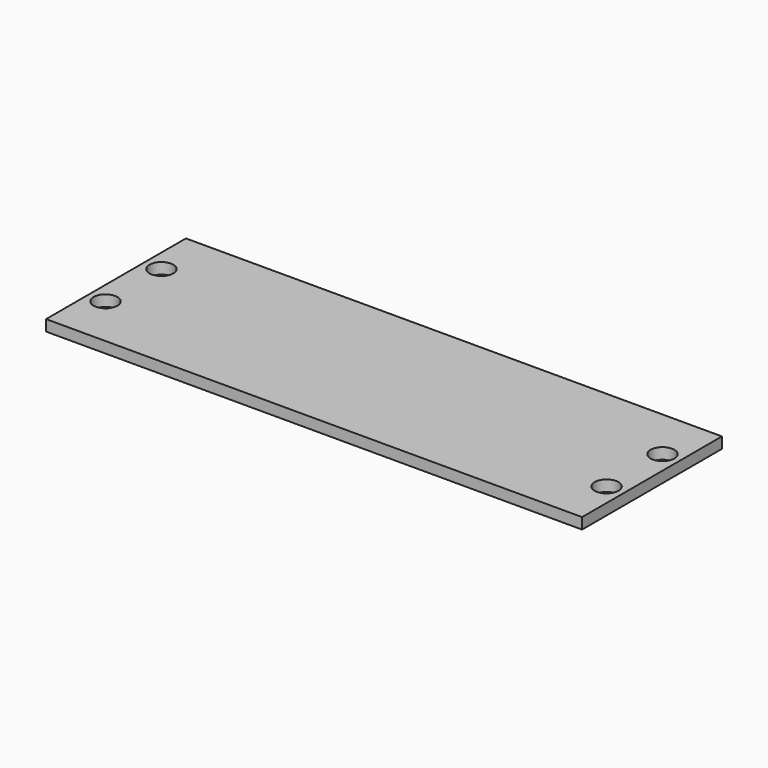
from build123d import *

# Parameters (mm, degrees)
F0_W     = 146.05
F0_H     = 47.625
F0_R     = 3.24
F1_DEPTH = 3


# Not quite as in the source:
# - ends of sketch curves that miss each other by under 0.0002 mm in the source are joined


with BuildPart() as f1:
    # F0 (on Top) → F1 (new body)
    with BuildSketch(Plane.XY):
        Rectangle(F0_W, F0_H)
        with Locations((-68.262, -9.5245)):
            Circle(F0_R, mode=Mode.SUBTRACT)
        with Locations((68.262, -9.5245)):
            Circle(F0_R, mode=Mode.SUBTRACT)
        with Locations((-68.262, 9.5245)):
            Circle(F0_R, mode=Mode.SUBTRACT)
        with BuildLine():
            Line((72.225, -15.859485), (72.225, -23.0125))
            Line((72.225, -23.0125), (-72.225, -23.0125))
            Line((-72.225, -23.0125), (-72.225, -15.874133))
            Line((-72.225, -15.874133), (-68.193705, -15.874133))
            ThreePointArc((-68.193705, -15.874133), (-61.912367271, -9.4562050029), (-68.3302949971, -3.174867271))
            Line((-68.3302949971, -3.174867271), (-72.225, -3.174867))
            Line((-72.225, -3.174867), (-72.225, 3.1745))
            Line((-72.225, 3.1745), (-68.262, 3.1745))
            ThreePointArc((-68.262, 3.1745), (-61.912, 9.5245), (-68.262, 15.8745))
            Line((-68.262, 15.8745), (-72.225, 15.8745))
            Line((-72.225, 15.8745), (-72.225, 23.0125))
            Line((-72.225, 23.0125), (72.225, 23.0125))
            Line((72.225, 23.0125), (72.225, 15.8745))
            Line((72.225, 15.8745), (68.262, 15.8745))
            ThreePointArc((68.262, 15.8745), (61.912, 9.5245), (68.262, 3.1745))
            Line((68.262, 3.1745), (72.225, 3.1745))
            Line((72.225, 3.1745), (72.225, -3.189515))
            Line((72.225, -3.189515), (67.825573, -3.189515))
            ThreePointArc((67.825573, -3.189515), (61.9270152731, -9.9609269812), (68.6984269812, -15.8594847269))
            Line((68.6984269812, -15.8594847269), (72.225, -15.859485))
        make_face(mode=Mode.SUBTRACT)
        with Locations((68.262, 9.5245)):
            Circle(F0_R, mode=Mode.SUBTRACT)
        with BuildLine():
            Line((-72.225, -23.0125), (72.225, -23.0125))
            Line((72.225, -23.0125), (72.225, -15.859485))
            Line((72.225, -15.859485), (68.698427, -15.859485))
            ThreePointArc((68.698427, -15.859485), (61.9270152731, -9.9609269812), (67.8255730188, -3.1895152731))
            Line((67.8255730188, -3.1895152731), (72.225, -3.189515))
            Line((72.225, -3.189515), (72.225, 3.1745))
            Line((72.225, 3.1745), (68.262, 3.1745))
            ThreePointArc((68.262, 3.1745), (61.912, 9.5245), (68.262, 15.8745))
            Line((68.262, 15.8745), (72.225, 15.8745))
            Line((72.225, 15.8745), (72.225, 23.0125))
            Line((72.225, 23.0125), (-72.225, 23.0125))
            Line((-72.225, 23.0125), (-72.225, 15.8745))
            Line((-72.225, 15.8745), (-68.262, 15.8745))
            ThreePointArc((-68.262, 15.8745), (-61.912, 9.5245), (-68.262, 3.1745))
            Line((-68.262, 3.1745), (-72.225, 3.1745))
            Line((-72.225, 3.1745), (-72.225, -3.174867))
            Line((-72.225, -3.174867), (-68.330295, -3.174867))
            ThreePointArc((-68.330295, -3.174867), (-61.912367271, -9.4562050029), (-68.1937050029, -15.874132729))
            Line((-68.1937050029, -15.874132729), (-72.225, -15.874133))
            Line((-72.225, -15.874133), (-72.225, -23.0125))
        make_face()
    extrude(amount=-F1_DEPTH)


solid = f1.part
